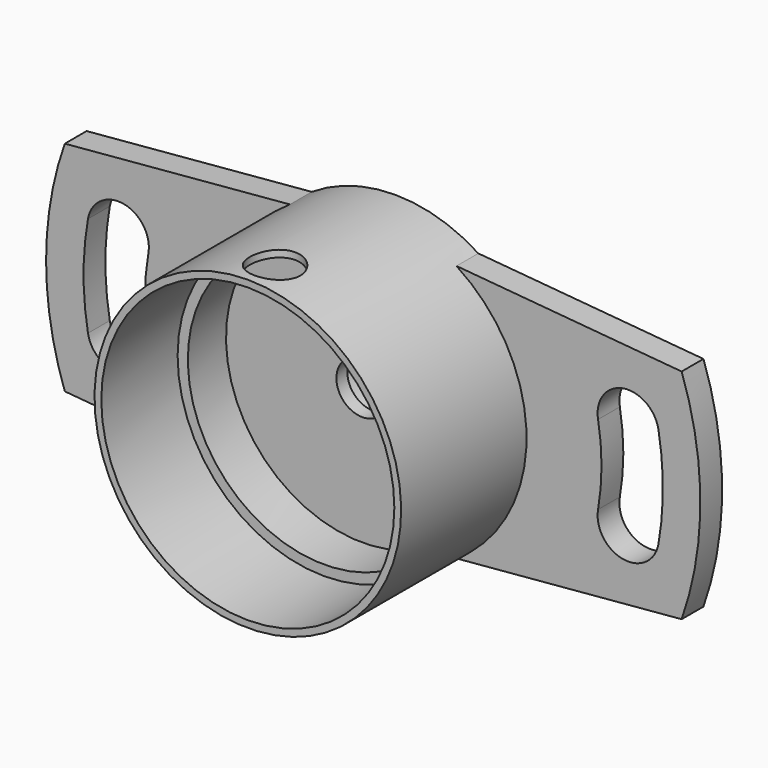
from build123d import *

# Parameters (mm, degrees)
F2_R     = 1.85
F3_DEPTH = 11.251
F4_R     = 4.7
F5_DEPTH = 2


with BuildPart() as f1:
    # F0 (on Right) → F1 (revolve)
    with BuildSketch(Plane.YZ):
        Polygon((11.5, 11.25), (0, 11.25), (0, 10.75), (7, 10.75), (7, 10), (10.5, 10), (10.5, 1.9), (11.5, 1.9), (11.5, 4), (19.5, 4), (19.5, 4.7), (11.5, 4.7), align=None)
    revolve(axis=Axis((0, 13.454885222, 0), (0, 1, 0)))

    # F2 (on Top) → F3 (cut, through all)
    with BuildSketch(Plane.XY):
        with Locations((0, 2.5)):
            Circle(F2_R)
    extrude(amount=F3_DEPTH, mode=Mode.SUBTRACT)

    # F4 (on face) → F5 (join)
    with BuildSketch(Plane(origin=(0, 11.5, 0), x_dir=(-1, 0, 0), z_dir=(0, 1, 0))):
        with BuildLine():
            ThreePointArc((22.627416998, -8), (23.6543654317, -4.0584474894), (24, 0))
            ThreePointArc((24, 0), (23.6543654317, 4.0584474894), (22.627416998, 8))
            Line((22.627416998, 8), (6.1119619567, 9.4449150891))
            ThreePointArc((6.1119619567, 9.4449150891), (9.88235984, 5.3760081839), (11.25, 0))
            ThreePointArc((11.25, 0), (9.88235984, -5.3760081839), (6.1119619567, -9.4449150891))
            Line((6.1119619567, -9.4449150891), (22.627416998, -8))
        make_face()
        with BuildLine():
            ThreePointArc((16.495529863, 2.9086069759), (18.3206389075, 5.5151328199), (20.9271647515, 3.6900237754))
            ThreePointArc((20.9271647515, 3.6900237754), (21.25, 0), (20.9271647515, -3.6900237754))
            ThreePointArc((20.9271647515, -3.6900237754), (18.3206389075, -5.5151328199), (16.495529863, -2.9086069759))
            ThreePointArc((16.495529863, -2.9086069759), (16.75, 0), (16.495529863, 2.9086069759))
        make_face(mode=Mode.SUBTRACT)
        with BuildLine():
            Line((-6.1119619567, 9.4449150891), (-22.627416998, 8))
            ThreePointArc((-22.627416998, 8), (-24, 0), (-22.627416998, -8))
            Line((-22.627416998, -8), (-6.1119619567, -9.4449150891))
            ThreePointArc((-6.1119619567, -9.4449150891), (-11.25, 0), (-6.1119619567, 9.4449150891))
        make_face()
        with BuildLine():
            ThreePointArc((-16.495529863, -2.9086069759), (-18.3206389075, -5.5151328199), (-20.9271647515, -3.6900237754))
            ThreePointArc((-20.9271647515, -3.6900237754), (-21.25, 0), (-20.9271647515, 3.6900237754))
            ThreePointArc((-20.9271647515, 3.6900237754), (-18.3206389075, 5.5151328199), (-16.495529863, 2.9086069759))
            ThreePointArc((-16.495529863, 2.9086069759), (-16.75, 0), (-16.495529863, -2.9086069759))
        make_face(mode=Mode.SUBTRACT)
        with BuildLine():
            ThreePointArc((11.25, 0), (9.88235984, 5.3760081839), (6.1119619567, 9.4449150891))
            ThreePointArc((6.1119619567, 9.4449150891), (0, 11.25), (-6.1119619567, 9.4449150891))
            ThreePointArc((-6.1119619567, 9.4449150891), (-11.25, 0), (-6.1119619567, -9.4449150891))
            ThreePointArc((-6.1119619567, -9.4449150891), (0, -11.25), (6.1119619567, -9.4449150891))
            ThreePointArc((6.1119619567, -9.4449150891), (9.88235984, -5.3760081839), (11.25, 0))
        make_face()
        Circle(F4_R, mode=Mode.SUBTRACT)
    extrude(amount=F5_DEPTH)


solid = f1.part
